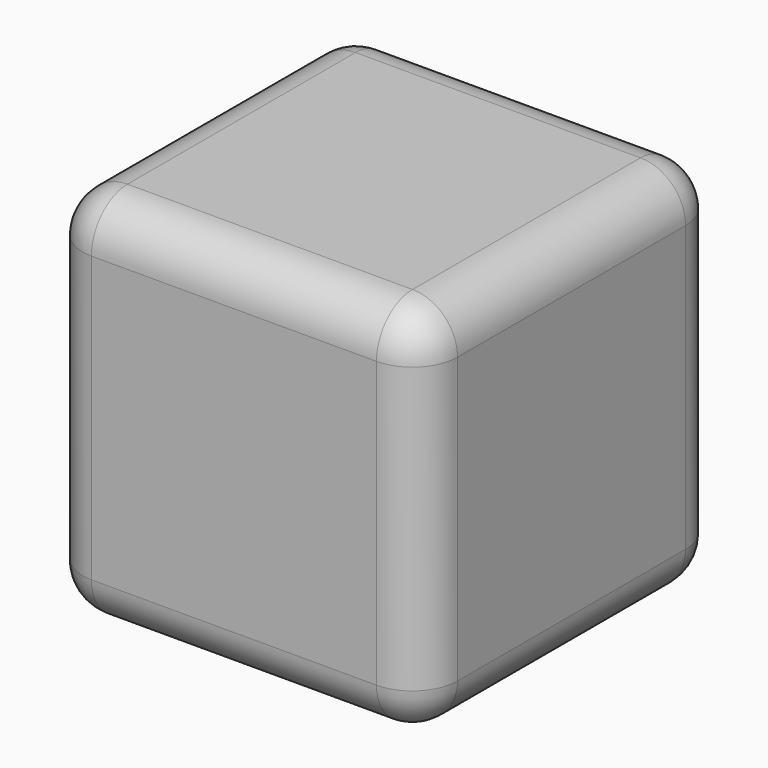
from build123d import *

# Parameters (mm, degrees)
F0_W         = 25
F0_H         = 25
F1_DEPTH     = 25
F2_R         = 3
F3_R         = 3
F4_R         = 3
F5_T1_DEPTH  = 19
F5_S5_W      = 3
F5_S5_H      = 3
F5_T6_DEPTH  = 3
F5_S11_W     = 3
F5_S11_H     = 3
F5_T12_DEPTH = 3
F5_S17_W     = 3
F5_S17_H     = 3
F5_T18_DEPTH = 3
F5_S23_W     = 3
F5_S23_H     = 3
F5_T24_DEPTH = 3


# Not quite as in the source:
# - a fillet or chamfer that OpenCascade refuses, or shapes differently, is made with other operations: its cross-section is extruded or revolved along the edge and cut away or added
# - a feature names something its author has since deleted; it is built from what else it names


with BuildPart() as f1:
    # F0 (on Top) → F1 (new body)
    with BuildSketch(Plane.XY):
        Rectangle(F0_W, F0_H)
    extrude(amount=F1_DEPTH)

    # F2
    f2_edges = [f1.edges().sort_by_distance(p)[0] for p in [
        (12.5, 0, 25),
    ]]
    fillet(f2_edges, radius=F2_R)

    # F3
    f3_edges = [f1.edges().sort_by_distance(p)[0] for p in [
        (-1.5, 12.5, 25),
        (9.5, 0, 25),
        (-12.5, 0, 25),
        (-1.5, -12.5, 25),
    ]]
    fillet(f3_edges, radius=F3_R)

    # F4
    f4_edges = [f1.edges().sort_by_distance(p)[0] for p in [
        (-1.5, 12.5, 0),
        (11.62132, 11.62132, 0),
        (-12.5, 0, 0),
        (12.5, 0, 0),
        (-1.5, -12.5, 0),
        (11.62132, -11.62132, 0),
    ]]
    fillet(f4_edges, radius=F4_R)

    # F5: fillet of radius 3 on 2 edges, made by hand

    # F5_s2 → F5_t1 (cut)
    with BuildSketch(Plane.XY.offset(3)):
        with BuildLine():
            ThreePointArc((-9.5, 12.5), (-11.6213203436, 11.6213203436), (-12.5, 9.5))
            Line((-12.5, 9.5), (-12.5, 12.5))
            Line((-12.5, 12.5), (-9.5, 12.5))
        make_face()
        with BuildLine():
            ThreePointArc((-12.5, -9.5), (-11.6213203436, -11.6213203436), (-9.5, -12.5))
            Line((-9.5, -12.5), (-12.5, -12.5))
            Line((-12.5, -12.5), (-12.5, -9.5))
        make_face()
    extrude(amount=F5_T1_DEPTH, mode=Mode.SUBTRACT)


with BuildPart() as f5_tool4:
    # F5_s5 → F5_t6 (new body)
    with BuildSketch(Plane.YZ.offset(-9.5)):
        with Locations((-11, 1.5)):
            Rectangle(F5_S5_W, F5_S5_H)
    extrude(amount=-F5_T6_DEPTH)

    # F5_s7 → F5_t8 (revolve, cut)
    with BuildSketch(Plane(origin=(-9.5, -9.5, 3), x_dir=(0, 0.7071067812, 0.7071067812), z_dir=(0, -0.7071067812, 0.7071067812))):
        with BuildLine():
            ThreePointArc((0, -3), (3, 0), (0, 3))
            Line((0, 3), (0, -3))
        make_face()
    revolve(axis=Axis((-9.5, -9.5, 3), (-1, 0, 0)), mode=Mode.SUBTRACT)


with BuildPart() as f1_1:
    add(f1.part)

    # F5_t3: cut F5_tool4
    add(f5_tool4.part, mode=Mode.SUBTRACT)


with BuildPart() as f5_tool10:
    # F5_s11 → F5_t12 (new body)
    with BuildSketch(Plane.YZ.offset(-9.5)):
        with Locations((-11, 23.5)):
            Rectangle(F5_S11_W, F5_S11_H)
    extrude(amount=-F5_T12_DEPTH)

    # F5_s13 → F5_t14 (revolve, cut)
    with BuildSketch(Plane(origin=(-9.5, -9.5, 22), x_dir=(0, 0.7071067812, -0.7071067812), z_dir=(0, 0.7071067812, 0.7071067812))):
        with BuildLine():
            ThreePointArc((0, -3), (3, 0), (0, 3))
            Line((0, 3), (0, -3))
        make_face()
    revolve(axis=Axis((-9.5, -9.5, 22), (-1, 0, 0)), mode=Mode.SUBTRACT)


with BuildPart() as f1_2:
    add(f1_1.part)

    # F5_t9: cut F5_tool10
    add(f5_tool10.part, mode=Mode.SUBTRACT)


with BuildPart() as f5_tool16:
    # F5_s17 → F5_t18 (new body)
    with BuildSketch(Plane.XZ.offset(-9.5)):
        with Locations((-11, 1.5)):
            Rectangle(F5_S17_W, F5_S17_H)
    extrude(amount=-F5_T18_DEPTH)

    # F5_s19 → F5_t20 (revolve, cut)
    with BuildSketch(Plane(origin=(-9.5, 9.5, 3), x_dir=(0.7071067812, 0, 0.7071067812), z_dir=(-0.7071067812, 0, 0.7071067812))):
        with BuildLine():
            ThreePointArc((0, -3), (3, 0), (0, 3))
            Line((0, 3), (0, -3))
        make_face()
    revolve(axis=Axis((-9.5, 9.5, 3), (0, 1, 0)), mode=Mode.SUBTRACT)


with BuildPart() as f1_3:
    add(f1_2.part)

    # F5_t15: cut F5_tool16
    add(f5_tool16.part, mode=Mode.SUBTRACT)


with BuildPart() as f5_tool22:
    # F5_s23 → F5_t24 (new body)
    with BuildSketch(Plane.XZ.offset(-9.5)):
        with Locations((-11, 23.5)):
            Rectangle(F5_S23_W, F5_S23_H)
    extrude(amount=-F5_T24_DEPTH)

    # F5_s25 → F5_t26 (revolve, cut)
    with BuildSketch(Plane(origin=(-9.5, 9.5, 22), x_dir=(0.7071067812, 0, -0.7071067812), z_dir=(0.7071067812, 0, 0.7071067812))):
        with BuildLine():
            ThreePointArc((0, -3), (3, 0), (0, 3))
            Line((0, 3), (0, -3))
        make_face()
    revolve(axis=Axis((-9.5, 9.5, 22), (0, 1, 0)), mode=Mode.SUBTRACT)


with BuildPart() as f1_4:
    add(f1_3.part)

    # F5_t21: cut F5_tool22
    add(f5_tool22.part, mode=Mode.SUBTRACT)


solid = f1_4.part
